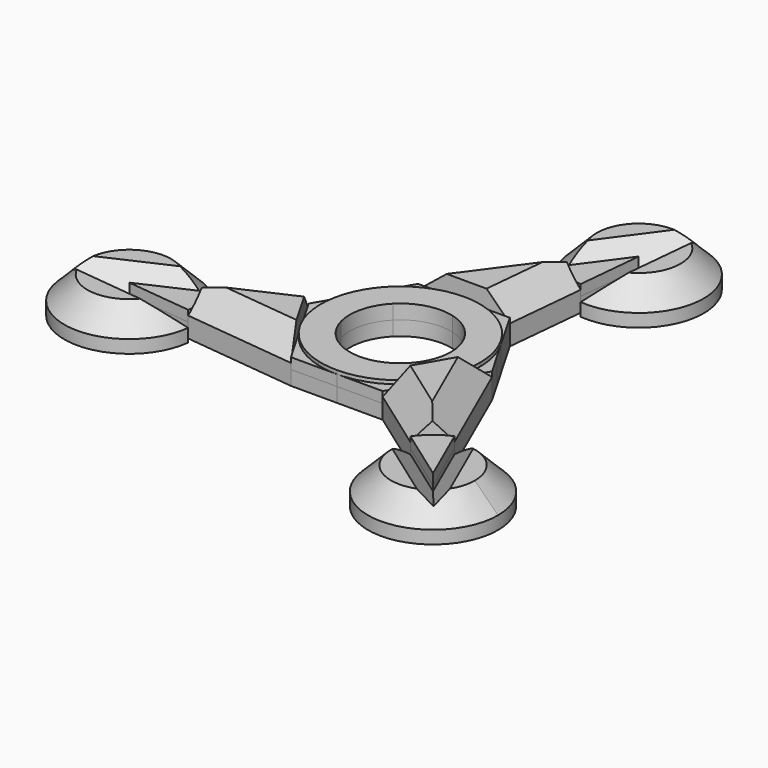
from build123d import *

# Parameters (mm, degrees)
F1_DEPTH       = 3.175
F1_DEPTH_BACK  = 3.175
F2_DEPTH       = 2.38125
F2_DEPTH_BACK  = 3.175
F3_DEPTH       = 6.35
F3_DEPTH_BACK  = 3.175
F4_DEPTH       = 3.96875
F4_DEPTH_BACK  = 3.96875
F5_DEPTH       = 2.38125
F5_DEPTH_BACK  = 3.175
F6_T1_DEPTH    = 51.0658567028
F6_T3_DEPTH    = 43.5956947451
F6_2_T1_DEPTH  = 43.5956947451
F6_2_T3_DEPTH  = 51.0658567028
F6_3_T1_DEPTH  = 43.5956947451
F6_3_T3_DEPTH  = 51.0658567028
F6_4_T4_DEPTH  = 40.4157991577
F6_4_T9_DEPTH  = 40.4157991577
F6_4_T12_ANGLE = 359.64
F6_4_T17_DEPTH = 40.4157991577
F6_4_T21_DEPTH = 40.4157991577
F6_5_T2_ANGLE  = 359.64
F6_5_T6_DEPTH  = 40.4157991577
F6_5_T11_DEPTH = 40.4157991577
F6_5_T17_DEPTH = 40.4157991577
F6_5_T21_DEPTH = 40.4157991577
F6_6_T2_ANGLE  = 268.0514708104
F6_6_T4_ANGLE  = 166.1085533485
F6_6_T8_DEPTH  = 40.4157991577
F6_6_T13_DEPTH = 40.4157991577
F6_6_T19_DEPTH = 40.4157991577
F6_6_T23_DEPTH = 40.4157991577


# Not quite as in the source:
# - a fillet or chamfer that OpenCascade refuses, or shapes differently, is made with other operations: its cross-section is extruded or revolved along the edge and cut away or added
# - a length typed as a fraction of an inch, garbled in the dataset ("3 / 203.2 mm" for 3/8 in), is restored


with BuildPart() as f1:
    # F0 (on Top) → F1 (new body, two sides)
    with BuildSketch(Plane.XY) as f1_sk:
        with BuildLine():
            Line((-4.5196275751, -16.8674797416), (-2.8761266387, -10.7338507446))
            ThreePointArc((-2.8761266387, -10.7338507446), (-7.8577241059, -7.8577241059), (-10.7338507446, -2.8761266387))
            Line((-10.7338507446, -2.8761266387), (-16.8674797416, -4.5196275751))
            ThreePointArc((-16.8674797416, -4.5196275751), (-16.1332463557, -6.6826093913), (-15.1229686637, -8.7312499131))
            ThreePointArc((-15.1229686637, -8.7312499131), (-10.6304964939, -13.8539326743), (-4.5196275751, -16.8674797416))
        make_face()
        with BuildLine():
            ThreePointArc((-7.8577241059, 7.8577241059), (-2.8761266387, 10.7338507446), (2.8761266387, 10.7338507446))
            Line((2.8761266387, 10.7338507446), (4.5196275751, 16.8674797416))
            ThreePointArc((4.5196275751, 16.8674797416), (2.2793136316, 17.3131058917), (0, 17.4625))
            ThreePointArc((0, 17.4625), (-6.6826094377, 16.1332463365), (-12.3478521665, 12.3478521665))
            Line((-12.3478521665, 12.3478521665), (-7.8577241059, 7.8577241059))
        make_face()
        with BuildLine():
            ThreePointArc((-10.7338507446, -2.8761266387), (-10.7338507446, 2.8761266387), (-7.8577241059, 7.8577241059))
            Line((-7.8577241059, 7.8577241059), (-12.3478521665, 12.3478521665))
            ThreePointArc((-12.3478521665, 12.3478521665), (-13.8539326905, 10.6304964728), (-15.12296859, 8.7312500408))
            ThreePointArc((-15.12296859, 8.7312500408), (-17.3131058887, 2.279313655), (-16.8674797416, -4.5196275751))
            Line((-16.8674797416, -4.5196275751), (-10.7338507446, -2.8761266387))
        make_face()
        with BuildLine():
            ThreePointArc((2.8761266387, 10.7338507446), (7.8577241059, 7.8577241059), (10.7338507446, 2.8761266387))
            Line((10.7338507446, 2.8761266387), (16.8674797416, 4.5196275751))
            ThreePointArc((16.8674797416, 4.5196275751), (16.1332463692, 6.6826093587), (15.122968699, 8.731249852))
            ThreePointArc((15.122968699, 8.731249852), (10.6304965218, 13.8539326528), (4.5196275751, 16.8674797416))
            Line((4.5196275751, 16.8674797416), (2.8761266387, 10.7338507446))
        make_face()
        with BuildLine():
            ThreePointArc((10.7338507446, 2.8761266387), (11.017431022, 1.450472311), (11.1125, 0))
            ThreePointArc((11.1125, 0), (10.266611305, -4.2525696422), (7.8577241059, -7.8577241059))
            Line((7.8577241059, -7.8577241059), (12.3478521665, -12.3478521665))
            ThreePointArc((12.3478521665, -12.3478521665), (13.853932765, -10.6304963756), (15.1229687125, -8.7312498287))
            ThreePointArc((15.1229687125, -8.7312498287), (16.8674797672, -4.5196274796), (17.4625, 0))
            ThreePointArc((17.4625, 0), (17.3131058917, 2.2793136316), (16.8674797416, 4.5196275751))
            Line((16.8674797416, 4.5196275751), (10.7338507446, 2.8761266387))
        make_face()
        with BuildLine():
            Line((12.3478521665, -12.3478521665), (7.8577241059, -7.8577241059))
            ThreePointArc((7.8577241059, -7.8577241059), (2.8761266387, -10.7338507446), (-2.8761266387, -10.7338507446))
            Line((-2.8761266387, -10.7338507446), (-4.5196275751, -16.8674797416))
            ThreePointArc((-4.5196275751, -16.8674797416), (-2.2793136142, -17.313105894), (3.53e-08, -17.4625))
            ThreePointArc((3.53e-08, -17.4625), (6.682609454, -16.1332463297), (12.3478521665, -12.3478521665))
        make_face()
    extrude(amount=-F1_DEPTH)
    extrude(f1_sk.sketch, amount=F1_DEPTH_BACK)

    # F0 (on Top) → F2 (join, two sides)
    with BuildSketch(Plane.XY) as f2_sk:
        with BuildLine():
            Line((4.6790627728, 17.4625), (4.5196275751, 16.8674797416))
            ThreePointArc((4.5196275751, 16.8674797416), (10.6304965218, 13.8539326528), (15.122968699, 8.731249852))
            Line((15.122968699, 8.731249852), (10.0819790757, 17.4625))
            Line((10.0819790757, 17.4625), (4.6790627728, 17.4625))
        make_face()
        with BuildLine():
            Line((17.4625, 4.6790627728), (16.8674797416, 4.5196275751))
            ThreePointArc((16.8674797416, 4.5196275751), (17.3131058917, 2.2793136316), (17.4625, 0))
            ThreePointArc((17.4625, 0), (16.8674797672, -4.5196274796), (15.1229687125, -8.7312498287))
            Line((15.1229687125, -8.7312498287), (20.1639581514, 0))
            Line((20.1639581514, 0), (17.4625, 4.6790627728))
        make_face()
        with BuildLine():
            Line((12.7834372272, -12.7834372272), (12.3478521665, -12.3478521665))
            ThreePointArc((12.3478521665, -12.3478521665), (6.682609454, -16.1332463297), (3.53e-08, -17.4625))
            Line((3.53e-08, -17.4625), (10.0819790757, -17.4625))
            Line((10.0819790757, -17.4625), (12.7834372272, -12.7834372272))
        make_face()
        with BuildLine():
            Line((-4.6790627728, -17.4625), (-4.5196275751, -16.8674797416))
            ThreePointArc((-4.5196275751, -16.8674797416), (-10.6304964939, -13.8539326743), (-15.1229686637, -8.7312499131))
            Line((-15.1229686637, -8.7312499131), (-10.0819790757, -17.4625))
            Line((-10.0819790757, -17.4625), (-4.6790627728, -17.4625))
        make_face()
        with BuildLine():
            Line((-17.4625, -4.6790627728), (-16.8674797416, -4.5196275751))
            ThreePointArc((-16.8674797416, -4.5196275751), (-17.3131058887, 2.279313655), (-15.12296859, 8.7312500408))
            Line((-15.12296859, 8.7312500408), (-20.1639581514, 0))
            Line((-20.1639581514, 0), (-17.4625, -4.6790627728))
        make_face()
        with BuildLine():
            Line((-12.7834372272, 12.7834372272), (-12.3478521665, 12.3478521665))
            ThreePointArc((-12.3478521665, 12.3478521665), (-6.6826094377, 16.1332463365), (0, 17.4625))
            Line((0, 17.4625), (-10.0819790757, 17.4625))
            Line((-10.0819790757, 17.4625), (-12.7834372272, 12.7834372272))
        make_face()
        with BuildLine():
            ThreePointArc((-15.12296859, 8.7312500408), (-13.8539326905, 10.6304964728), (-12.3478521665, 12.3478521665))
            Line((-12.3478521665, 12.3478521665), (-12.7834372272, 12.7834372272))
            Line((-12.7834372272, 12.7834372272), (-15.12296859, 8.7312500408))
        make_face()
        with BuildLine():
            ThreePointArc((-15.1229686637, -8.7312499131), (-16.1332463557, -6.6826093913), (-16.8674797416, -4.5196275751))
            Line((-16.8674797416, -4.5196275751), (-17.4625, -4.6790627728))
            Line((-17.4625, -4.6790627728), (-15.1229686637, -8.7312499131))
        make_face()
        with BuildLine():
            ThreePointArc((3.53e-08, -17.4625), (-2.2793136142, -17.313105894), (-4.5196275751, -16.8674797416))
            Line((-4.5196275751, -16.8674797416), (-4.6790627728, -17.4625))
            Line((-4.6790627728, -17.4625), (3.53e-08, -17.4625))
        make_face()
        with BuildLine():
            ThreePointArc((15.1229687125, -8.7312498287), (13.853932765, -10.6304963756), (12.3478521665, -12.3478521665))
            Line((12.3478521665, -12.3478521665), (12.7834372272, -12.7834372272))
            Line((12.7834372272, -12.7834372272), (15.1229687125, -8.7312498287))
        make_face()
        with BuildLine():
            ThreePointArc((15.122968699, 8.731249852), (16.1332463692, 6.6826093587), (16.8674797416, 4.5196275751))
            Line((16.8674797416, 4.5196275751), (17.4625, 4.6790627728))
            Line((17.4625, 4.6790627728), (15.122968699, 8.731249852))
        make_face()
        with BuildLine():
            ThreePointArc((0, 17.4625), (2.2793136316, 17.3131058917), (4.5196275751, 16.8674797416))
            Line((4.5196275751, 16.8674797416), (4.6790627728, 17.4625))
            Line((4.6790627728, 17.4625), (0, 17.4625))
        make_face()
    extrude(amount=F2_DEPTH)
    extrude(f2_sk.sketch, amount=-F2_DEPTH_BACK)


with BuildPart() as f3:
    # F0 (on Top) → F3 (new body, two sides)
    with BuildSketch(Plane.XY) as f3_sk:
        with BuildLine():
            Line((25.8182363481, -25.8182363481), (12.7834372272, -12.7834372272))
            Line((12.7834372272, -12.7834372272), (10.0819790757, -17.4625))
            Line((10.0819790757, -17.4625), (24.2952466492, -27.6159690372))
            ThreePointArc((24.2952466492, -27.6159690372), (25.0196206528, -26.6856549328), (25.8182363481, -25.8182363481))
        make_face()
        with BuildLine():
            Line((20.1639581514, 0), (15.1229687125, -8.7312498287))
            Line((15.1229687125, -8.7312498287), (12.7834372272, -12.7834372272))
            Line((12.7834372272, -12.7834372272), (25.8182363481, -25.8182363481))
            ThreePointArc((25.8182363481, -25.8182363481), (27.8608858867, -24.1241256529), (30.1816043452, -22.8369993881))
            Line((30.1816043452, -22.8369993881), (20.1639581514, 0))
        make_face()
    extrude(amount=F3_DEPTH)
    extrude(f3_sk.sketch, amount=-F3_DEPTH_BACK)

    # F6: chamfer of 5.08 on 2 edges, made by hand

    # F6_s2 → F6_t1 (cut)
    with BuildSketch(Plane(origin=(18.5194987555, -42.2184786293, 0), x_dir=(0, 0, 1), z_dir=(-0.4017091961, 0.9157672858, 0))):
        Polygon((1.27, 18.4654932278), (6.35, 13.3854932278), (6.35, 18.4654932278), align=None)
    extrude(amount=F6_T1_DEPTH, mode=Mode.SUBTRACT)

    # F6_s4 → F6_t3 (cut)
    with BuildSketch(Plane(origin=(4.3046564772, -3.0750983918, 0), x_dir=(0, 0, 1), z_dir=(0.8137027356, -0.5812812211, 0))):
        Polygon((1.27, 8.348818912), (6.35, 3.268818912), (6.35, 8.348818912), align=None)
    extrude(amount=F6_T3_DEPTH, mode=Mode.SUBTRACT)


with BuildPart() as f3b:
    # F0 (on Top) → F3, piece 2 (new body, two sides)
    with BuildSketch(Plane.XY) as f3_2_sk:
        with BuildLine():
            Line((9.4501303843, 35.2683667324), (4.6790627728, 17.4625))
            Line((4.6790627728, 17.4625), (10.0819790757, 17.4625))
            Line((10.0819790757, 17.4625), (11.7685074117, 34.848285308))
            ThreePointArc((11.7685074117, 34.848285308), (10.600644762, 35.0104545447), (9.4501303843, 35.2683667324))
        make_face()
        with BuildLine():
            Line((-10.0819790757, 17.4625), (0, 17.4625))
            Line((0, 17.4625), (4.6790627728, 17.4625))
            Line((4.6790627728, 17.4625), (9.4501303843, 35.2683667324))
            ThreePointArc((9.4501303843, 35.2683667324), (6.9616627161, 36.1902977763), (4.6866194437, 37.556535784))
            Line((4.6866194437, 37.556535784), (-10.0819790757, 17.4625))
        make_face()
    extrude(amount=F3_DEPTH)
    extrude(f3_2_sk.sketch, amount=-F3_DEPTH_BACK)

    # F6#2: chamfer of 5.08 on 2 edges, made by hand

    # F6_2_s2 → F6_2_t1 (cut)
    with BuildSketch(Plane(origin=(0.5107850878, 5.2654910597, 0), x_dir=(0, 0, 1), z_dir=(0.0965529364, 0.9953278507, 0))):
        Polygon((6.35, 3.268818912), (1.27, 8.348818912), (6.35, 8.348818912), align=None)
    extrude(amount=F6_2_T1_DEPTH, mode=Mode.SUBTRACT)

    # F6_2_s4 → F6_2_t3 (cut)
    with BuildSketch(Plane(origin=(27.3025256244, 37.1475957023, 0), x_dir=(0, 0, 1), z_dir=(-0.5922231354, -0.8057740117, 0))):
        Polygon((1.27, 18.4654932278), (6.35, 13.3854932278), (6.35, 18.4654932278), align=None)
    extrude(amount=F6_2_T3_DEPTH, mode=Mode.SUBTRACT)


with BuildPart() as f3c:
    # F0 (on Top) → F3, piece 3 (new body, two sides)
    with BuildSketch(Plane.XY) as f3_3_sk:
        with BuildLine():
            Line((-10.0819790757, -17.4625), (-15.1229686637, -8.7312499131))
            Line((-15.1229686637, -8.7312499131), (-17.4625, -4.6790627728))
            Line((-17.4625, -4.6790627728), (-35.2683667324, -9.4501303843))
            ThreePointArc((-35.2683667324, -9.4501303843), (-34.9037635186, -11.2831145199), (-34.7815319755, -13.1480074912))
            ThreePointArc((-34.7815319755, -13.1480074912), (-34.8032213919, -13.9349666021), (-34.8682237889, -14.7195363959))
            Line((-34.8682237889, -14.7195363959), (-10.0819790757, -17.4625))
        make_face()
        with BuildLine():
            Line((-35.2683667324, -9.4501303843), (-17.4625, -4.6790627728))
            Line((-17.4625, -4.6790627728), (-20.1639581514, 0))
            Line((-20.1639581514, 0), (-36.0637540609, -7.2323162708))
            ThreePointArc((-36.0637540609, -7.2323162708), (-35.6202654148, -8.324799612), (-35.2683667324, -9.4501303843))
        make_face()
    extrude(amount=F3_DEPTH)
    extrude(f3_3_sk.sketch, amount=-F3_DEPTH_BACK)

    # F6#3: chamfer of 5.08 on 2 edges, made by hand

    # F6_3_s2 → F6_3_t1 (cut)
    with BuildSketch(Plane(origin=(-4.815441565, -2.1903926679, 0), x_dir=(0, 0, 1), z_dir=(-0.9102556721, -0.4140466296, 0))):
        Polygon((1.27, 8.348818912), (6.35, 3.268818912), (6.35, 8.348818912), align=None)
    extrude(amount=F6_3_T1_DEPTH, mode=Mode.SUBTRACT)

    # F6_3_s4 → F6_3_t3 (cut)
    with BuildSketch(Plane(origin=(-45.8220243799, 5.070882927, 0), x_dir=(0, 0, 1), z_dir=(0.9939323315, -0.1099932742, 0))):
        Polygon((1.27, 18.4654932278), (6.35, 13.3854932278), (6.35, 18.4654932278), align=None)
    extrude(amount=F6_3_T3_DEPTH, mode=Mode.SUBTRACT)


with BuildPart() as f4:
    # F0 (on Top) → F4 (new body, two sides)
    with BuildSketch(Plane.XY) as f4_sk:
        with BuildLine():
            Line((13.1480074912, 49.0690319755), (11.7685074117, 34.848285308))
            ThreePointArc((11.7685074117, 34.848285308), (22.7506906804, 38.4897535588), (27.4355074912, 49.0690319755))
            ThreePointArc((27.4355074912, 49.0690319755), (6.6966287811, 61.8170659019), (4.6866194437, 37.556535784))
            Line((4.6866194437, 37.556535784), (13.1480074912, 49.0690319755))
        make_face()
    extrude(amount=F4_DEPTH)
    extrude(f4_sk.sketch, amount=-F4_DEPTH_BACK)

    # F6#4: chamfer of 5.08 on 3 edges, made by hand


with BuildPart() as f4b:
    # F0 (on Top) → F4, piece 2 (new body, two sides)
    with BuildSketch(Plane.XY) as f4_2_sk:
        with BuildLine():
            ThreePointArc((-36.0637540609, -7.2323162708), (-63.1778021748, -15.4008411988), (-34.8682237889, -14.7195363959))
            Line((-34.8682237889, -14.7195363959), (-49.0690319755, -13.1480074912))
            Line((-49.0690319755, -13.1480074912), (-36.0637540609, -7.2323162708))
        make_face()
    extrude(amount=F4_DEPTH)
    extrude(f4_2_sk.sketch, amount=-F4_DEPTH_BACK)

    # F6#5: chamfer of 5.08 on 3 edges, made by hand

    # F6_5_s1 → F6_5_t2 (revolve, cut)
    with BuildSketch(Plane(origin=(0.8179896941, -5.0214395273, 0), x_dir=(0, 0, 1), z_dir=(0.1607801593, -0.9869902433, 0))):
        Polygon((-1.11125, 36.2570945471), (3.96875, 41.3370945471), (3.96875, 36.2570945471), align=None)
    revolve(axis=Axis((-49.0690319755, -13.1480074912, 3.96875), (0, 0, 1)), revolution_arc=F6_5_T2_ANGLE, mode=Mode.SUBTRACT)


with BuildPart() as f4c:
    # F0 (on Top) → F4, piece 3 (new body, two sides)
    with BuildSketch(Plane.XY) as f4_3_sk:
        with BuildLine():
            ThreePointArc((50.2085244843, -35.9210244843), (43.7354563578, -23.9599496687), (30.1816043452, -22.8369993881))
            Line((30.1816043452, -22.8369993881), (35.9210244843, -35.9210244843))
            Line((35.9210244843, -35.9210244843), (24.2952466492, -27.6159690372))
            ThreePointArc((24.2952466492, -27.6159690372), (31.5604422163, -49.526831279), (50.2085244843, -35.9210244843))
        make_face()
    extrude(amount=F4_DEPTH)
    extrude(f4_3_sk.sketch, amount=-F4_DEPTH_BACK)

    # F6#6: chamfer of 5.08 on 4 edges, made by hand

    # F6_6_s1 → F6_6_t2 (revolve, cut)
    with BuildSketch(Plane(origin=(34.6588261556, 1.1791406399, 0), x_dir=(0, 0, 1), z_dir=(0.9994217752, 0.0340016949, 0))):
        Polygon((-1.11125, 22.8341297711), (3.96875, 27.9141297711), (3.96875, 22.8341297711), align=None)
    revolve(axis=Axis((35.9210244843, -35.9210244843, 3.96875), (0, 0, 1)), revolution_arc=F6_6_T2_ANGLE, mode=Mode.SUBTRACT)

    # F6_6_s3 → F6_6_t4 (revolve, cut)
    with BuildSketch(Plane.XZ.offset(35.9210244843)):
        Polygon((45.1285244843, 3.96875), (50.2085244843, -1.11125), (50.2085244843, 3.96875), align=None)
    revolve(axis=Axis((35.9210244843, -35.9210244843, 3.96875), (0, 0, 1)), revolution_arc=F6_6_T4_ANGLE, mode=Mode.SUBTRACT)


with BuildPart() as f5:
    # F0 (on Top) → F5 (new body, two sides)
    with BuildSketch(Plane.XY) as f5_sk:
        with BuildLine():
            Line((35.9210244843, -35.9210244843), (25.8182363481, -25.8182363481))
            ThreePointArc((25.8182363481, -25.8182363481), (25.0196206528, -26.6856549328), (24.2952466492, -27.6159690372))
            Line((24.2952466492, -27.6159690372), (35.9210244843, -35.9210244843))
        make_face()
        with BuildLine():
            ThreePointArc((30.1816043452, -22.8369993881), (27.8608858867, -24.1241256529), (25.8182363481, -25.8182363481))
            Line((25.8182363481, -25.8182363481), (35.9210244843, -35.9210244843))
            Line((35.9210244843, -35.9210244843), (30.1816043452, -22.8369993881))
        make_face()
    extrude(amount=F5_DEPTH)
    extrude(f5_sk.sketch, amount=-F5_DEPTH_BACK)


with BuildPart() as f5b:
    # F0 (on Top) → F5, piece 2 (new body, two sides)
    with BuildSketch(Plane.XY) as f5_2_sk:
        with BuildLine():
            Line((13.1480074912, 49.0690319755), (9.4501303843, 35.2683667324))
            ThreePointArc((9.4501303843, 35.2683667324), (10.600644762, 35.0104545447), (11.7685074117, 34.848285308))
            Line((11.7685074117, 34.848285308), (13.1480074912, 49.0690319755))
        make_face()
        with BuildLine():
            ThreePointArc((4.6866194437, 37.556535784), (6.9616627161, 36.1902977763), (9.4501303843, 35.2683667324))
            Line((9.4501303843, 35.2683667324), (13.1480074912, 49.0690319755))
            Line((13.1480074912, 49.0690319755), (4.6866194437, 37.556535784))
        make_face()
    extrude(amount=F5_DEPTH)
    extrude(f5_2_sk.sketch, amount=-F5_DEPTH_BACK)


with BuildPart() as f5c:
    # F0 (on Top) → F5, piece 3 (new body, two sides)
    with BuildSketch(Plane.XY) as f5_3_sk:
        with BuildLine():
            Line((-49.0690319755, -13.1480074912), (-35.2683667324, -9.4501303843))
            ThreePointArc((-35.2683667324, -9.4501303843), (-35.6202654148, -8.324799612), (-36.0637540609, -7.2323162708))
            Line((-36.0637540609, -7.2323162708), (-49.0690319755, -13.1480074912))
        make_face()
        with BuildLine():
            ThreePointArc((-34.7815319755, -13.1480074912), (-34.9037635186, -11.2831145199), (-35.2683667324, -9.4501303843))
            Line((-35.2683667324, -9.4501303843), (-49.0690319755, -13.1480074912))
            Line((-49.0690319755, -13.1480074912), (-34.8682237889, -14.7195363959))
            ThreePointArc((-34.8682237889, -14.7195363959), (-34.8032213919, -13.9349666021), (-34.7815319755, -13.1480074912))
        make_face()
    extrude(amount=F5_DEPTH)
    extrude(f5_3_sk.sketch, amount=-F5_DEPTH_BACK)


with BuildPart() as f6_4_tool2:
    # F6_4_s3 → F6_4_t4 (new body)
    with BuildSketch(Plane(origin=(11.8287423736, 16.0940912723, 0), x_dir=(0, 0, 1), z_dir=(0.5922231354, 0.8057740117, 0))):
        Polygon((-1.11125, -18.4654932278), (3.96875, -23.5454932278), (3.96875, -18.4654932278), align=None)
    extrude(amount=F6_4_T4_DEPTH)

    split(bisect_by=Plane(origin=(8.3098119839, -0.8061029818, 0), x_dir=(0, 0, 1), z_dir=(-0.9953278507, 0.0965529364, 0)), keep=Keep.TOP)


with BuildPart() as f4_1:
    add(f4.part)

    # F6_4_t1: cut F6_4_tool2
    add(f6_4_tool2.part, mode=Mode.SUBTRACT)


with BuildPart() as f6_4_tool7:
    # F6_4_s8 → F6_4_t9 (new body)
    with BuildSketch(Plane(origin=(6.0995775113, 62.8782468794, 0), x_dir=(0, 0, 1), z_dir=(-0.0965529364, -0.9953278507, 0))):
        Polygon((-1.11125, -8.348818912), (3.96875, -13.428818912), (3.96875, -8.348818912), align=None)
    extrude(amount=F6_4_T9_DEPTH)

    split(bisect_by=Plane(origin=(-14.8790145553, 10.9356922967, 0), x_dir=(0, 0, 1), z_dir=(0.8057740117, -0.5922231354, 0)), keep=Keep.TOP)


with BuildPart() as f4_2:
    add(f4_1.part)

    # F6_4_t6: cut F6_4_tool7
    add(f6_4_tool7.part, mode=Mode.SUBTRACT)

    # F6_4_s11 → F6_4_t12 (revolve, cut)
    with BuildSketch(Plane(origin=(-5.042448021, 1.9465092507, 0), x_dir=(0, 0, 1), z_dir=(0.9329044068, -0.3601241005, 0))):
        Polygon((3.96875, -41.3041305388), (-1.11125, -36.2241305388), (3.96875, -36.2241305388), align=None)
    revolve(axis=Axis((13.1480074912, 49.0690319755, 3.96875), (0, 0, -1)), revolution_arc=F6_4_T12_ANGLE, mode=Mode.SUBTRACT)


with BuildPart() as f6_4_tool15:
    # F6_4_s16 → F6_4_t17 (new body)
    with BuildSketch(Plane(origin=(11.8287423736, 16.0940912723, 0), x_dir=(0, 0, 1), z_dir=(0.5922231354, 0.8057740117, 0))):
        Polygon((-1.11125, -18.4654932278), (3.96875, -23.5454932278), (3.96875, -18.4654932278), align=None)
    extrude(amount=F6_4_T17_DEPTH)

    split(bisect_by=Plane(origin=(8.3098119839, -0.8061029818, 0), x_dir=(0, 0, 1), z_dir=(0.9953278507, -0.0965529364, 0)), keep=Keep.TOP)


with BuildPart() as f6_4_tool19:
    # F6_4_s20 → F6_4_t21 (new body)
    with BuildSketch(Plane(origin=(6.0995775113, 62.8782468794, 0), x_dir=(0, 0, 1), z_dir=(-0.0965529364, -0.9953278507, 0))):
        Polygon((-1.11125, -8.348818912), (3.96875, -13.428818912), (3.96875, -8.348818912), align=None)
    extrude(amount=F6_4_T21_DEPTH)

    split(bisect_by=Plane(origin=(-14.8790145553, 10.9356922967, 0), x_dir=(0, 0, 1), z_dir=(-0.8057740117, 0.5922231354, 0)), keep=Keep.TOP)


with BuildPart() as f6_4_tool15_1:
    add(f6_4_tool15.part)

    # F6_4_t23: intersect F6_4_tool19
    add(f6_4_tool19.part, mode=Mode.INTERSECT)


with BuildPart() as f4_3:
    add(f4_2.part)

    # F6_4_t13: cut F6_4_tool15
    add(f6_4_tool15_1.part, mode=Mode.SUBTRACT)


with BuildPart() as f6_5_tool4:
    # F6_5_s5 → F6_5_t6 (new body)
    with BuildSketch(Plane(origin=(-19.8522630794, 2.1969457542, 0), x_dir=(0, 0, 1), z_dir=(-0.9939323315, 0.1099932742, 0))):
        Polygon((-1.11125, -18.4654932278), (3.96875, -23.5454932278), (3.96875, -18.4654932278), align=None)
    extrude(amount=F6_5_T6_DEPTH)

    split(bisect_by=Plane(origin=(-3.4568003316, 7.5995597696, 0), x_dir=(0, 0, 1), z_dir=(0.4140466296, -0.9102556721, 0)), keep=Keep.TOP)


with BuildPart() as f4b_1:
    add(f4b.part)

    # F6_5_t3: cut F6_5_tool4
    add(f6_5_tool4.part, mode=Mode.SUBTRACT)


with BuildPart() as f6_5_tool9:
    # F6_5_s10 → F6_5_t11 (new body)
    with BuildSketch(Plane(origin=(-57.5039478986, -26.1567343626, 0), x_dir=(0, 0, 1), z_dir=(0.9102556721, 0.4140466296, 0))):
        Polygon((3.96875, -13.428818912), (-1.11125, -8.348818912), (3.96875, -8.348818912), align=None)
    extrude(amount=F6_5_T11_DEPTH)

    split(bisect_by=Plane(origin=(-2.0310800592, -18.3534507365, 0), x_dir=(0, 0, 1), z_dir=(0.1099932742, 0.9939323315, 0)), keep=Keep.TOP)


with BuildPart() as f4b_2:
    add(f4b_1.part)

    # F6_5_t8: cut F6_5_tool9
    add(f6_5_tool9.part, mode=Mode.SUBTRACT)


with BuildPart() as f6_5_tool15:
    # F6_5_s16 → F6_5_t17 (new body)
    with BuildSketch(Plane(origin=(-19.8522630794, 2.1969457542, 0), x_dir=(0, 0, 1), z_dir=(-0.9939323315, 0.1099932742, 0))):
        Polygon((-1.11125, -18.4654932278), (3.96875, -23.5454932278), (3.96875, -18.4654932278), align=None)
    extrude(amount=F6_5_T17_DEPTH)

    split(bisect_by=Plane(origin=(-3.4568003316, 7.5995597696, 0), x_dir=(0, 0, 1), z_dir=(-0.4140466296, 0.9102556721, 0)), keep=Keep.TOP)


with BuildPart() as f6_5_tool19:
    # F6_5_s20 → F6_5_t21 (new body)
    with BuildSketch(Plane(origin=(-57.5039478986, -26.1567343626, 0), x_dir=(0, 0, 1), z_dir=(0.9102556721, 0.4140466296, 0))):
        Polygon((3.96875, -13.428818912), (-1.11125, -8.348818912), (3.96875, -8.348818912), align=None)
    extrude(amount=F6_5_T21_DEPTH)

    split(bisect_by=Plane(origin=(-2.0310800592, -18.3534507365, 0), x_dir=(0, 0, 1), z_dir=(-0.1099932742, -0.9939323315, 0)), keep=Keep.TOP)


with BuildPart() as f6_5_tool15_1:
    add(f6_5_tool15.part)

    # F6_5_t23: intersect F6_5_tool19
    add(f6_5_tool19.part, mode=Mode.INTERSECT)


with BuildPart() as f4b_3:
    add(f4b_2.part)

    # F6_5_t13: cut F6_5_tool15
    add(f6_5_tool15_1.part, mode=Mode.SUBTRACT)


with BuildPart() as f6_6_tool6:
    # F6_6_s7 → F6_6_t8 (new body)
    with BuildSketch(Plane(origin=(8.0235207058, -18.2910370265, 0), x_dir=(0, 0, 1), z_dir=(0.4017091961, -0.9157672858, 0))):
        Polygon((3.96875, -23.5454932278), (-1.11125, -18.4654932278), (3.96875, -18.4654932278), align=None)
    extrude(amount=F6_6_T8_DEPTH)

    split(bisect_by=Plane(origin=(-4.8530116523, -6.7934567878, 0), x_dir=(0, 0, 1), z_dir=(0.5812812211, 0.8137027356, 0)), keep=Keep.TOP)


with BuildPart() as f4c_1:
    add(f4c.part)

    # F6_6_t5: cut F6_6_tool6
    add(f6_6_tool6.part, mode=Mode.SUBTRACT)


with BuildPart() as f6_6_tool11:
    # F6_6_s12 → F6_6_t13 (new body)
    with BuildSketch(Plane(origin=(51.4043703873, -36.7215125168, 0), x_dir=(0, 0, 1), z_dir=(-0.8137027356, 0.5812812211, 0))):
        Polygon((-1.11125, -8.348818912), (3.96875, -13.428818912), (3.96875, -8.348818912), align=None)
    extrude(amount=F6_6_T13_DEPTH)

    split(bisect_by=Plane(origin=(16.9100946145, 7.4177584398, 0), x_dir=(0, 0, 1), z_dir=(-0.9157672858, -0.4017091961, 0)), keep=Keep.TOP)


with BuildPart() as f4c_2:
    add(f4c_1.part)

    # F6_6_t10: cut F6_6_tool11
    add(f6_6_tool11.part, mode=Mode.SUBTRACT)


with BuildPart() as f6_6_tool17:
    # F6_6_s18 → F6_6_t19 (new body)
    with BuildSketch(Plane(origin=(51.4043703873, -36.7215125168, 0), x_dir=(0, 0, 1), z_dir=(-0.8137027356, 0.5812812211, 0))):
        Polygon((-1.11125, -8.348818912), (3.96875, -13.428818912), (3.96875, -8.348818912), align=None)
    extrude(amount=F6_6_T19_DEPTH)

    split(bisect_by=Plane(origin=(16.9100946145, 7.4177584398, 0), x_dir=(0, 0, 1), z_dir=(0.9157672858, 0.4017091961, 0)), keep=Keep.TOP)


with BuildPart() as f6_6_tool21:
    # F6_6_s22 → F6_6_t23 (new body)
    with BuildSketch(Plane(origin=(8.0235207058, -18.2910370265, 0), x_dir=(0, 0, 1), z_dir=(0.4017091961, -0.9157672858, 0))):
        Polygon((3.96875, -23.5454932278), (-1.11125, -18.4654932278), (3.96875, -18.4654932278), align=None)
    extrude(amount=F6_6_T23_DEPTH)

    split(bisect_by=Plane(origin=(-4.8530116523, -6.7934567878, 0), x_dir=(0, 0, 1), z_dir=(-0.5812812211, -0.8137027356, 0)), keep=Keep.TOP)


with BuildPart() as f6_6_tool17_1:
    add(f6_6_tool17.part)

    # F6_6_t25: intersect F6_6_tool21
    add(f6_6_tool21.part, mode=Mode.INTERSECT)


with BuildPart() as f4c_3:
    add(f4c_2.part)

    # F6_6_t15: cut F6_6_tool17
    add(f6_6_tool17_1.part, mode=Mode.SUBTRACT)


solid = Compound([f1.part, f3.part, f3b.part, f3c.part, f5.part, f5b.part, f5c.part, f4_3.part, f4b_3.part, f4c_3.part])
